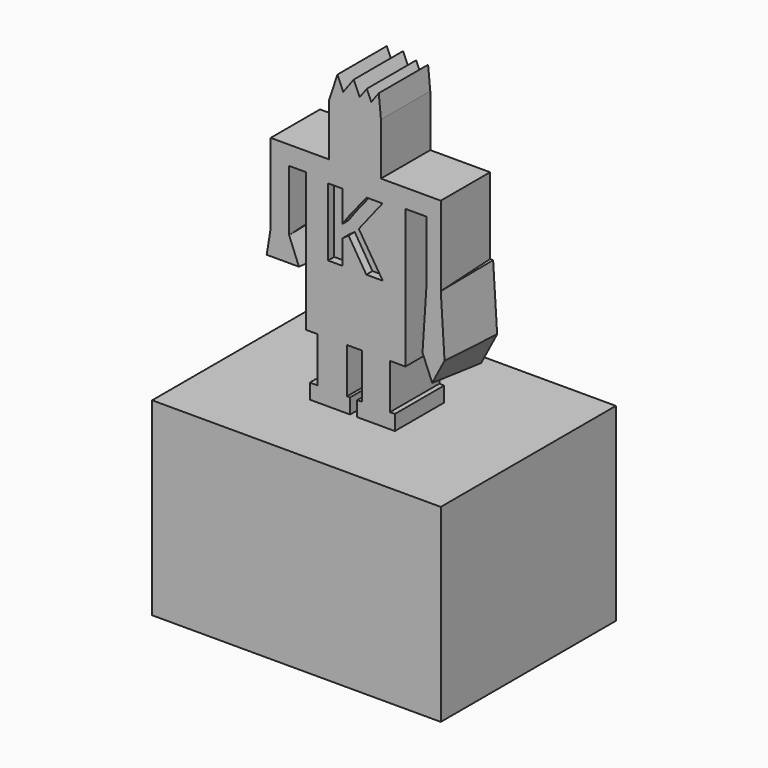
from build123d import *

# Parameters (mm, degrees)
F0_W         = 21.393219009
F0_H         = 21.393219009
F0_W_2       = 12.0918184984
F0_H_2       = 18.6101384461
F1_DEPTH     = 25.4
F3_DEPTH     = 25.4
F3_TAPER     = -3
F4_W         = 118.9088746905
F4_H         = 90.1495143771
F5_DEPTH     = 77.978
F6_TEXT_SIZE = 39.2139824625
F7_DEPTH     = 3.175


# Not quite as in the source:
# - a length typed as a fraction of an inch, garbled in the dataset ("3 / 203.2 mm" for 3/8 in), is restored
# - Text() gives the source's letters only with a copy of the font that has no kerning and outlines rounded to 1/6400 em; it was checked with that copy


with BuildPart() as f1:
    # F0 (on Front) → F1 (new body)
    with BuildSketch(Plane.XZ):
        Polygon((-10.1883225143, 37.3318567872), (-19.6337904781, 37.3318567872), (-19.6337904781, 29.6352189034), (-19.6337904781, -27.5610499084), (-14.839021489, -27.5610499084), (-2.7472029906, -27.5610499084), (3.4537302563, -27.5610499084), (9.6546635032, -27.5610499084), (14.9254556745, -27.5610499084), (21.2929844856, -27.5610499084), (21.2929844856, 29.6352189034), (21.2929844856, 37.3318567872), (11.2048964947, 37.3318567872), align=None)
        Polygon((-19.6337904781, 29.6352189034), (-19.6337904781, 37.3318567872), (-34.216940403, 37.3318567872), (-34.216940403, 4.5214416459), (-26.6207940876, 4.5214416459), (-26.6207940876, 29.6352189034), align=None)
        with Locations((0.5082869902, 48.0284662917)):
            Rectangle(F0_W, F0_H)
        Polygon((-6.7289518192, 69.2252442241), (-10.1883225143, 58.7250757962), (11.2048964947, 58.7250757962), (10.3208585018, 68.0196038684), (7.2195872795, 63.7965960196), (5.3896177806, 68.0196038684), (2.4291200817, 63.9882876363), (0, 69.5939511061), (-4.3323384598, 63.6945962906), align=None)
        Polygon((35.8536057174, 37.3318567872), (21.2929844856, 37.3318567872), (21.2929844856, 29.6352189034), (29.9627184868, 29.6352189034), (29.9627184868, 4.5214416459), (35.8536057174, 4.5214416459), align=None)
        with Locations((-8.7931122398, -36.8661191314)):
            Rectangle(F0_W_2, F0_H_2)
        Polygon((-2.7472029906, -46.1711883545), (-14.839021489, -46.1711883545), (-18.0945117027, -46.1711883545), (-18.0945117027, -52.3721203208), (-1.5070163645, -52.3721203208), (-1.5070163645, -46.1711883545), align=None)
        Polygon((9.6546635032, -27.5610499084), (3.4537302563, -27.5610499084), (3.4537302563, -46.1711883545), (14.9254556745, -46.1711883545), (14.9254556745, -27.5610499084), align=None)
        Polygon((14.9254556745, -46.1711883545), (3.4537302563, -46.1711883545), (1.4384266688, -46.1711883545), (1.4384266688, -52.3721203208), (16.9407594949, -52.3721203208), (16.9407594949, -46.1711883545), align=None)
    extrude(amount=F1_DEPTH)

    # F2 (on face) → F3 (join)
    with BuildSketch(Plane.XZ.offset(25.4)):
        Polygon((32.3183760047, 2.3330994882), (29.9627184868, 4.5214416459), (28.3295959234, -20.2069189399), (32.3183760047, -29.9253277481), (37.4061278999, -20.2069189399), (35.8536057174, 4.5214416459), align=None)
        Polygon((-26.6207940876, 4.5214416459), (-34.216940403, 4.5214416459), (-35.8570180833, -5.6228227913), (-22.5834678859, -5.6228227913), align=None)
        Polygon((35.8536057174, 4.5214416459), (29.9627184868, 4.5214416459), (32.3183760047, 2.3330994882), align=None)
    extrude(amount=-F3_DEPTH, taper=F3_TAPER)

    # F4 (on face) → F5 (join)
    with BuildSketch(Plane(origin=(0, 0, -52.3721203208), x_dir=(1, 0, 0), z_dir=(0, 0, -1))):
        with Locations((2.0279027522, 12.3517736793)):
            Rectangle(F4_W, F4_H)
    extrude(amount=F5_DEPTH)

    # F6 (on face) → F7 (cut)
    with BuildSketch(Plane.XZ.offset(25.4)):
        with Locations((-14.1170332208, 0.534363091)):
            Text('K', F6_TEXT_SIZE, font='Open Sans', font_style=FontStyle.BOLD, text_align=(TextAlign.LEFT, TextAlign.BOTTOM))
    extrude(amount=-F7_DEPTH, mode=Mode.SUBTRACT)


solid = f1.part
